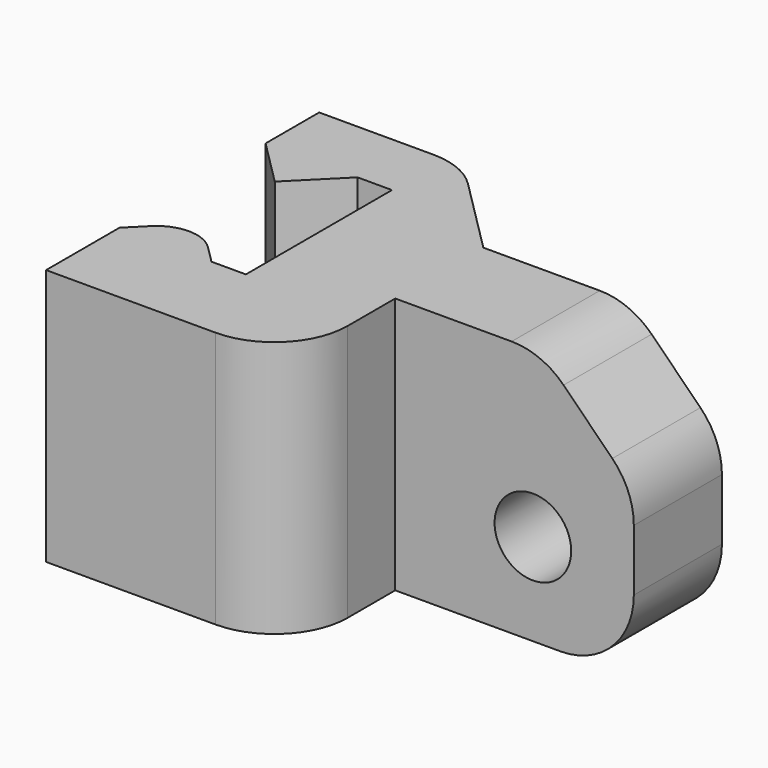
from build123d import *

# Parameters (mm, degrees)
F1_DEPTH = 17.78
F2_W     = 7.62
F2_H     = 17.78
F3_DEPTH = 16.51
F4_SIZE  = 6.35
F5_R     = 2.65
F6_DEPTH = 25.4
F7_R     = 2.794
F8_R     = 5.08
F9_R     = 5.08
F10_R    = 5.08
F11_R    = 5.08


# Not quite as in the source:
# - a feature names something its author has since deleted; it is built from what else it names


with BuildPart() as f1:
    # F0 (on Top) → F1 (new body)
    with BuildSketch(Plane.XY):
        Polygon((5.5632305153, 1.0289779667), (5.5632305153, -11.6080572072), (3.1819805153, -11.6080572072), (0, -8.4260766918), (-3.1819805153, -11.6080572072), (-3.1819805153, -17.9580572072), (13.6277864288, -17.9580572072), (13.6277864288, -1.148290263), (6.8148051953, 5.6646909705), (-0.4051948047, 5.6646909705), (-3.1819805153, 5.6646909705), (-3.1819805153, 1.0289779667), (0, -2.1530025487), (3.1819805153, 1.0289779667), align=None)
    extrude(amount=F1_DEPTH)

    # F2 (on face) → F3 (join)
    with BuildSketch(Plane.YZ.offset(13.6277864288)):
        with Locations((-4.958290263, 8.89)):
            Rectangle(F2_W, F2_H)
    extrude(amount=F3_DEPTH)

    # F4
    f4_edges = [f1.edges().sort_by_distance(p)[0] for p in [
        (30.137786, -4.95829, 17.78),
    ]]
    chamfer(f4_edges, length=F4_SIZE)

    # F5 (on face) → F6 (cut)
    with BuildSketch(Plane.XZ.offset(8.768290263)):
        with Locations((23.1527864288, 6.35)):
            Circle(F5_R)
    extrude(amount=-F6_DEPTH, mode=Mode.SUBTRACT)

    # F7
    f7_edges = [f1.edges().sort_by_distance(p)[0] for p in [
        (0, -8.426077, 8.89),
    ]]
    fillet(f7_edges, radius=F7_R)

    # F8
    f8_edges = [f1.edges().sort_by_distance(p)[0] for p in [
        (6.814805, 5.664691, 8.89),
    ]]
    fillet(f8_edges, radius=F8_R)

    # F9
    f9_edges = [f1.edges().sort_by_distance(p)[0] for p in [
        (30.137786, -4.95829, 0),
    ]]
    fillet(f9_edges, radius=F9_R)

    # F10
    f10_edges = [f1.edges().sort_by_distance(p)[0] for p in [
        (13.627786, -17.958057, 8.89),
    ]]
    fillet(f10_edges, radius=F10_R)

    # F11
    f11_edges = [f1.edges().sort_by_distance(p)[0] for p in [
        (30.137786, -4.95829, 11.43),
        (23.787786, -4.95829, 17.78),
    ]]
    fillet(f11_edges, radius=F11_R)


solid = f1.part
